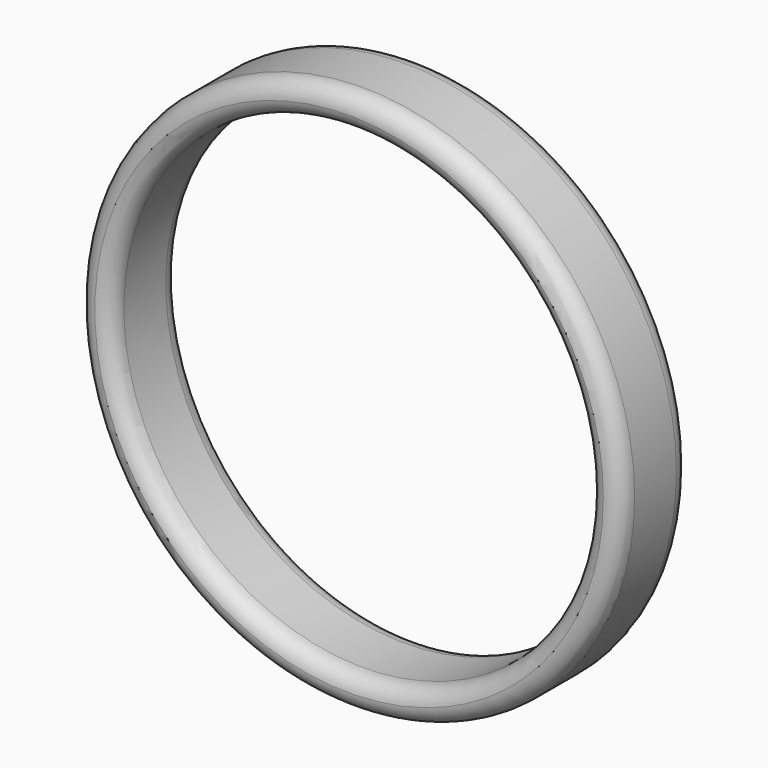
from build123d import *

# Parameters (mm, degrees)
F0_R     = 7.9375
F0_R_2   = 6.985
F1_DEPTH = 2.54
F2_R     = 0.508


# Not quite as in the source:
# - a fillet or chamfer that OpenCascade refuses, or shapes differently, is made with other operations: its cross-section is extruded or revolved along the edge and cut away or added


with BuildPart() as f1:
    # F0 (on Front) → F1 (new body)
    with BuildSketch(Plane.XZ):
        Circle(F0_R)
        Circle(F0_R_2, mode=Mode.SUBTRACT)
    extrude(amount=F1_DEPTH)

    # F2
    f2_edges = [f1.edges().sort_by_distance(p)[0] for p in [
        (-7.9375, -2.54, 0),
        (-7.9375, 0, 0),
    ]]
    fillet(f2_edges, radius=F2_R)

    # F3: fillet of radius 0.508 on 2 edges, made by hand

    # F3_s1 → F3_t2 (revolve, cut)
    with BuildSketch(Plane.XY):
        with BuildLine():
            ThreePointArc((7.4295, 0), (7.112, -0.1680052083), (6.985, -0.5040156248))
            Line((6.985, -0.5040156248), (6.985, 0))
            Line((6.985, 0), (7.4295, 0))
        make_face()
    revolve(axis=Axis((0, 0, 0), (0, -1, 0)), mode=Mode.SUBTRACT)

    # F3_s3 → F3_t4 (revolve, cut)
    with BuildSketch(Plane.XY):
        with BuildLine():
            ThreePointArc((7.4295, -2.54), (7.112, -2.3719947917), (6.985, -2.0359843752))
            Line((6.985, -2.0359843752), (6.985, -2.54))
            Line((6.985, -2.54), (7.4295, -2.54))
        make_face()
    revolve(axis=Axis((0, -2.54, 0), (0, -1, 0)), mode=Mode.SUBTRACT)


solid = f1.part
